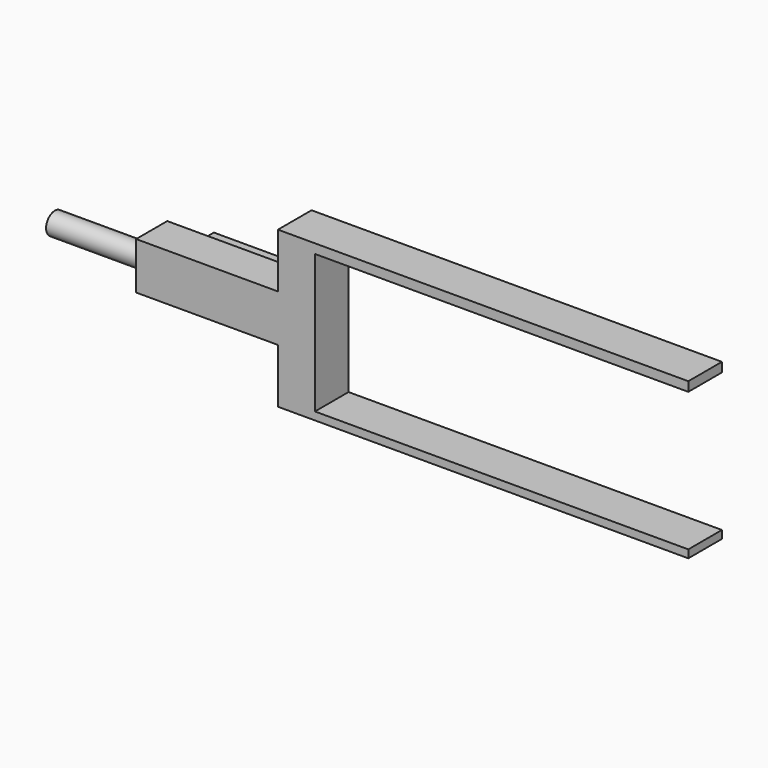
from build123d import *

# Parameters (mm, degrees)
F0_W      = 59.395711869
F0_H      = 250.2426505089
F1_DEPTH  = 67.4364492297
F2_R      = 17.4264129212
F3_DEPTH  = 222.8358983994
F4_W      = 62.507584691
F4_H      = 75.5731239915
F5_DEPTH  = 227.648139
F6_W      = 115.2810156345
F6_H      = 19.8185071349
F7_DEPTH  = 53.9569482207
F8_W      = 67.4364492297
F8_H      = 12.6657411456
F8_H_2    = 15.0272101164
F9_DEPTH  = 599.2090702057
F10_R     = 17.5883740648
F11_DEPTH = 151.8874019384
F12_R     = 10.9031193455
F13_DEPTH = 69.4709941745


# Not quite as in the source:
# - a feature names something its author has since deleted; it is built from what else it names


with BuildPart() as f1:
    # F0 (on Front) → F1 (new body)
    with BuildSketch(Plane.XZ):
        Rectangle(F0_W, F0_H)
    extrude(amount=F1_DEPTH)

    # F2 (on face) → F3 (join)
    with BuildSketch(Plane.XY.offset(125.1213252544)):
        with Locations((0, -33.2162864506)):
            Circle(F2_R)
    extrude(amount=-F3_DEPTH)

    # F4 (on face) → F5 (join)
    with BuildSketch(Plane(origin=(-29.6978559345, 0, 0), x_dir=(0, -1, 0), z_dir=(-1, 0, 0))):
        with Locations((36.1826568842, 0)):
            Rectangle(F4_W, F4_H)
    extrude(amount=F5_DEPTH)

    # F6 (on face) → F7 (join)
    with BuildSketch(Plane(origin=(0, -4.9288645387, 0), x_dir=(-1, 0, 0), z_dir=(0, 1, 0))):
        with Locations((168.05139184, 0)):
            Rectangle(F6_W, F6_H)
    extrude(amount=F7_DEPTH)

    # F8 (on face) → F9 (join)
    with BuildSketch(Plane.YZ.offset(29.6978559345)):
        with Locations((-33.7182246149, -118.7884546816)):
            Rectangle(F8_W, F8_H)
        with Locations((-33.7182246149, 117.6077201962)):
            Rectangle(F8_W, F8_H_2)
    extrude(amount=F9_DEPTH)

    # F10 (on face) → F11 (join)
    with BuildSketch(Plane(origin=(-257.3459949344, 0, 0), x_dir=(0, -1, 0), z_dir=(-1, 0, 0))):
        with Locations((40.5630767345, 0)):
            Circle(F10_R)
    extrude(amount=F11_DEPTH)

    # F12 (on face) → F13 (join)
    with BuildSketch(Plane(origin=(0, 0, -9.9092535675), x_dir=(1, 0, 0), z_dir=(0, 0, -1))):
        with Locations((-176.2370765209, -20.2873200178)):
            Circle(F12_R)
    extrude(amount=F13_DEPTH)


solid = f1.part
